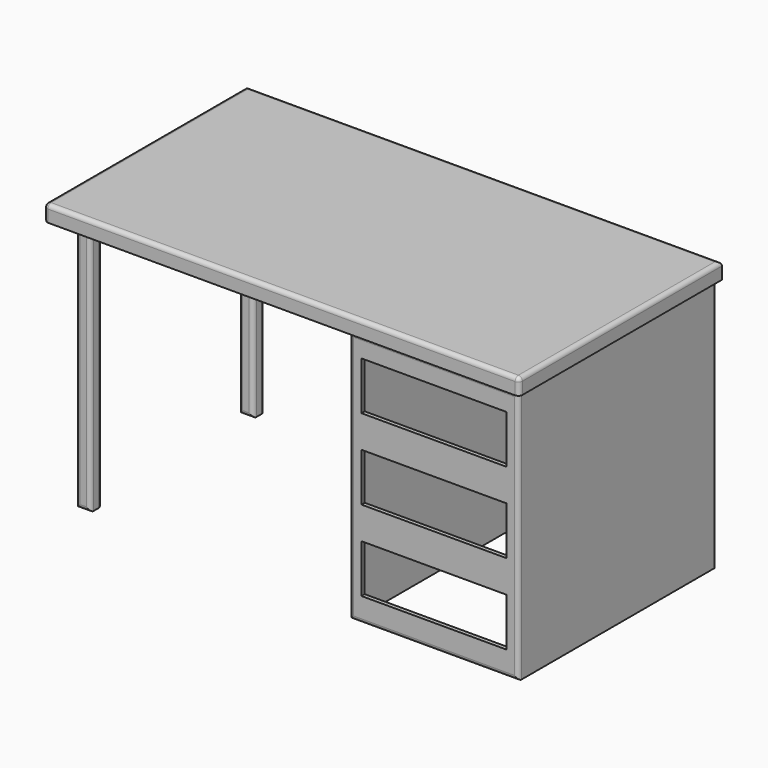
from build123d import *

# Parameters (mm, degrees)
F0_W     = 1500
F0_H     = 800
F1_DEPTH = 50.8
F2_W     = 45.72
F2_H     = 45.72
F3_DEPTH = 800
F4_W     = 533.4
F4_H     = 774.6
F4_W_2   = 508
F4_H_2   = 749.2
F5_DEPTH = 800
F6_R     = 12.69999
F6_2_R   = 12.69999
F6_3_R   = 12.69999
F6_4_R   = 12.69999
F7_W     = 457.2
F7_H     = 152.4
F8_DEPTH = 25.4


# Not quite as in the source:
# - a fillet or chamfer is up to 0.001 mm smaller than in the source, because OpenCascade refuses the exact size


with BuildPart() as f1:
    # F0 (on Top) → F1 (new body)
    with BuildSketch(Plane.XY):
        Rectangle(F0_W, F0_H)
    extrude(amount=F1_DEPTH)

    # F6#2 (radius 12.7 in the source; OpenCascade refuses exactly that, so slightly less here)
    f6_2_edges = [f1.edges().sort_by_distance(p)[0] for p in [
        (0, 400, 50.8),
        (-750, 0, 50.8),
        (0, -400, 50.8),
        (750, 0, 50.8),
        (-750, 0, 0),
        (-750, -400, 25.4),
        (750, -400, 25.4),
    ]]
    fillet(f6_2_edges, radius=F6_2_R)


with BuildPart() as f3:
    # F2 (on face) → F3 (new body)
    with BuildSketch(Plane(origin=(0, 0, 0), x_dir=(1, 0, 0), z_dir=(0, 0, -1))):
        with Locations((-671.26, 321.26)):
            Rectangle(F2_W, F2_H)
    extrude(amount=F3_DEPTH)

    # F6#3 (radius 12.7 in the source; OpenCascade refuses exactly that, so slightly less here)
    f6_3_edges = [f3.edges().sort_by_distance(p)[0] for p in [
        (-648.4, -344.12, -400),
        (-694.12, -344.12, -400),
        (-671.26, -344.12, 0),
        (-671.26, -344.12, -800),
        (-694.12, -298.4, -400),
        (-648.4, -298.4, -400),
        (-671.26, -298.4, 0),
        (-671.26, -298.4, -800),
    ]]
    fillet(f6_3_edges, radius=F6_3_R)


with BuildPart() as f3b:
    # F2 (on face) → F3, piece 2 (new body)
    with BuildSketch(Plane(origin=(0, 0, 0), x_dir=(1, 0, 0), z_dir=(0, 0, -1))):
        with Locations((-671.26, -321.26)):
            Rectangle(F2_W, F2_H)
    extrude(amount=F3_DEPTH)

    # F6#4 (radius 12.7 in the source; OpenCascade refuses exactly that, so slightly less here)
    f6_4_edges = [f3b.edges().sort_by_distance(p)[0] for p in [
        (-648.4, 298.4, -400),
        (-694.12, 298.4, -400),
        (-671.26, 298.4, 0),
        (-671.26, 298.4, -800),
        (-694.12, 344.12, -400),
        (-648.4, 344.12, -400),
        (-671.26, 344.12, 0),
        (-671.26, 344.12, -800),
    ]]
    fillet(f6_4_edges, radius=F6_4_R)


with BuildPart() as f5:
    # F4 (on face) → F5 (new body)
    with BuildSketch(Plane(origin=(0, 0, 0), x_dir=(1, 0, 0), z_dir=(0, 0, -1))):
        with Locations((470.6, 0)):
            Rectangle(F4_W, F4_H)
        with Locations((470.6, 0)):
            Rectangle(F4_W_2, F4_H_2, mode=Mode.SUBTRACT)
    extrude(amount=F5_DEPTH)

    # F6 (radius 12.7 in the source; OpenCascade refuses exactly that, so slightly less here)
    f6_edges = [f5.edges().sort_by_distance(p)[0] for p in [
        (737.3, -387.3, -400),
        (203.9, -387.3, -400),
        (470.6, -387.3, 0),
        (470.6, -387.3, -800),
    ]]
    fillet(f6_edges, radius=F6_R)

    # F7 (on face) → F8 (cut)
    with BuildSketch(Plane.XZ.offset(387.3)):
        with Locations((470.6, -139.7)):
            Rectangle(F7_W, F7_H)
        with Locations((470.6, -393.7)):
            Rectangle(F7_W, F7_H)
        with Locations((470.6, -647.7)):
            Rectangle(F7_W, F7_H)
    extrude(amount=-F8_DEPTH, mode=Mode.SUBTRACT)


solid = Compound([f1.part, f3.part, f3b.part, f5.part])
